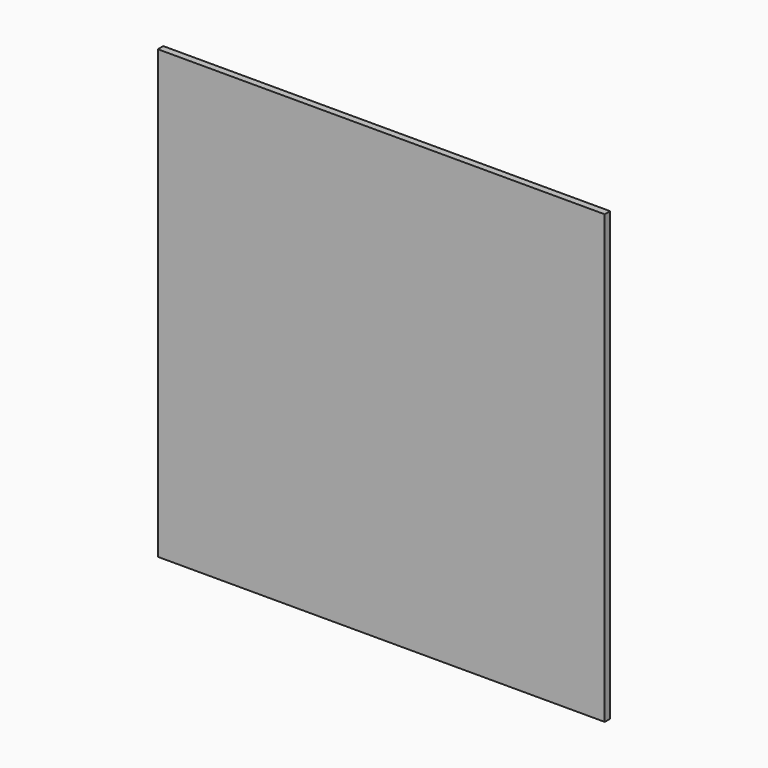
from build123d import *

# Parameters (mm, degrees)
F0_W     = 838.2
F0_H     = 838.2
F1_DEPTH = 12.7


# Not quite as in the source:
# - a length typed as a fraction of an inch, garbled in the dataset ("3 / 203.2 mm" for 3/8 in), is restored


with BuildPart() as f1:
    # F0 (on Front) → F1 (new body)
    with BuildSketch(Plane.XZ):
        with Locations((-4.1731838137, -27.9828987203)):
            Rectangle(F0_W, F0_H)
    extrude(amount=F1_DEPTH)


solid = f1.part
